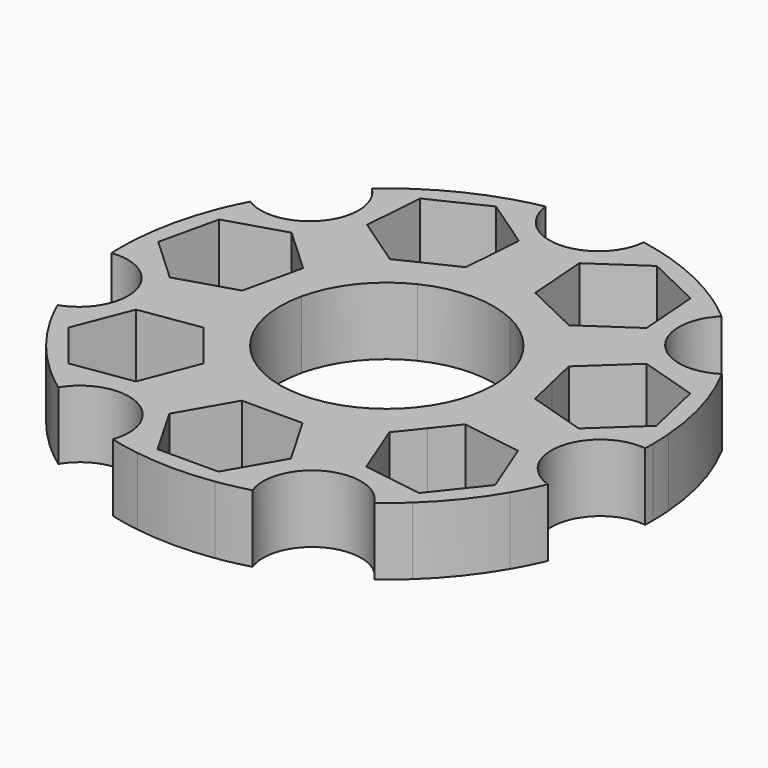
from build123d import *

# Parameters (mm, degrees)
F1_DEPTH = 6.9977
F4_D     = 10.16


# Not quite as in the source:
# - a feature names something its author has since deleted; it is built from what else it names


with BuildPart() as f1:
    # F0 (on Top) → F1 (new body)
    with BuildSketch(Plane.XY):
        with BuildLine():
            Line((13.000663339, 2.9673182751), (10.80089488, 2.4652351906))
            ThreePointArc((10.80089488, 2.4652351906), (11.0089999639, 1.2404170862), (11.0786603321, 0))
            ThreePointArc((11.0786603321, 0), (10.4569630833, -3.65904876), (8.6616464645, -6.9074304395))
            Line((8.6616464645, -6.9074304395), (10.4257240625, -8.3142349481))
            Line((10.4257240625, -8.3142349481), (12.9401280453, -5.1612711132))
            Line((12.9401280453, -5.1612711132), (20.9156255847, -6.3633827272))
            Line((20.9156255847, -6.3633827272), (23.8623151585, -13.8714220112))
            ThreePointArc((23.8623151585, -13.8714220112), (26.6500942722, -7.1832380314), (27.6012034762, 0))
            ThreePointArc((27.6012034762, 0), (27.5803414567, 1.0729391714), (27.5177869348, 2.1442564078))
            Line((27.5177869348, 2.1442564078), (21.6052967122, -3.3417341773))
            Line((21.6052967122, -3.3417341773), (13.8980443892, -0.9643627375))
            Line((13.8980443892, -0.9643627375), (13.000663339, 2.9673182751))
        make_face()
        with BuildLine():
            ThreePointArc((4.8068495738, 9.9815285367), (8.6616446562, 6.9074327071), (10.80089488, 2.4652351906))
            Line((10.80089488, 2.4652351906), (13.000663339, 2.9673182751))
            Line((13.000663339, 2.9673182751), (12.1032822888, 6.8989992876))
            Line((12.1032822888, 6.8989992876), (18.0157725115, 12.3849898727))
            Line((18.0157725115, 12.3849898727), (25.7230248345, 10.0076184329))
            ThreePointArc((25.7230248345, 10.0076184329), (21.5794879008, 17.2090713076), (15.4806129272, 22.8511937704))
            Line((15.4806129272, 22.8511937704), (16.0833555213, 14.8081635766))
            Line((16.0833555213, 14.8081635766), (9.419258347, 10.2646580813))
            Line((9.419258347, 10.2646580813), (5.7858384629, 12.0144204305))
            Line((5.7858384629, 12.0144204305), (4.8068495738, 9.9815285367))
        make_face()
        with BuildLine():
            Line((10.4257240625, -8.3142349481), (8.6616464645, -6.9074304395))
            ThreePointArc((8.6616464645, -6.9074304395), (4.8068513159, -9.9815276977), (0, -11.0786603321))
            Line((0, -11.0786603321), (0, -12.7))
            Line((0, -12.7), (0, -13.335))
            Line((0, -13.335), (4.0327916303, -13.335))
            Line((4.0327916303, -13.335), (8.0655832606, -20.32))
            Line((8.0655832606, -20.32), (4.0327916303, -27.305))
            ThreePointArc((4.0327916303, -27.305), (11.9757152285, -24.8678241529), (18.8335071928, -20.1773496811))
            Line((18.8335071928, -20.1773496811), (10.8580096534, -18.975238067))
            Line((10.8580096534, -18.975238067), (7.9113200797, -11.467198783))
            Line((7.9113200797, -11.467198783), (10.4257240625, -8.3142349481))
        make_face()
        with BuildLine():
            ThreePointArc((-4.8068513159, 9.9815276977), (-9.668e-07, 11.0786603321), (4.8068495738, 9.9815285367))
            Line((4.8068495738, 9.9815285367), (5.7858384629, 12.0144204305))
            Line((5.7858384629, 12.0144204305), (2.1524185788, 13.7641827798))
            Line((2.1524185788, 13.7641827798), (1.5496759847, 21.8072129736))
            Line((1.5496759847, 21.8072129736), (8.2137731589, 26.3507184689))
            ThreePointArc((8.2137731589, 26.3507184689), (-2.4087e-06, 27.6012034762), (-8.213777758, 26.3507170353))
            Line((-8.213777758, 26.3507170353), (-1.5496797908, 21.8072127031))
            Line((-1.5496797908, 21.8072127031), (-2.1524209811, 13.7641824041))
            Line((-2.1524209811, 13.7641824041), (-5.7858405598, 12.0144194207))
            Line((-5.7858405598, 12.0144194207), (-4.8068513159, 9.9815276977))
        make_face()
        Polygon((12.1032822888, 6.8989992876), (13.000663339, 2.9673182751), (13.8980443892, -0.9643627375), (21.6052967122, -3.3417341773), (27.5177869348, 2.1442564078), (25.7230248345, 10.0076184329), (18.0157725115, 12.3849898727), align=None)
        Polygon((15.188042256, 0.2325806629), (14.4864534349, 3.3064403636), (13.7848646139, 6.3803000643), (18.4073569698, 10.6693472491), (24.4330269677, 8.8106750325), (25.8362046098, 2.6629556311), (21.2137122539, -1.6260915537), align=None, mode=Mode.SUBTRACT)
        with BuildLine():
            Line((0, -12.7), (0, -11.0786603321))
            ThreePointArc((0, -11.0786603321), (-4.8068504449, -9.9815281172), (-8.661645259, -6.9074319513))
            Line((-8.661645259, -6.9074319513), (-10.4257226114, -8.3142367677))
            Line((-10.4257226114, -8.3142367677), (-7.9113180783, -11.4672001638))
            Line((-7.9113180783, -11.4672001638), (-10.8580063416, -18.9752399621))
            Line((-10.8580063416, -18.9752399621), (-18.8335036712, -20.1773529681))
            ThreePointArc((-18.8335036712, -20.1773529681), (-11.9757130584, -24.867825198), (-4.0327916303, -27.305))
            Line((-4.0327916303, -27.305), (-8.0655832606, -20.32))
            Line((-8.0655832606, -20.32), (-4.0327916303, -13.335))
            Line((-4.0327916303, -13.335), (0, -13.335))
            Line((0, -13.335), (0, -12.7))
        make_face()
        Polygon((12.9401280453, -5.1612711132), (10.4257240625, -8.3142349481), (7.9113200797, -11.467198783), (10.8580096534, -18.975238067), (18.8335071928, -20.1773496811), (23.8623151585, -13.8714220112), (20.9156255847, -6.3633827272), align=None)
        Polygon((9.6514286337, -11.7294776807), (11.6172353839, -9.2644332279), (13.5830421342, -6.7993887751), (19.8184311195, -7.7392214916), (22.1222066044, -13.6091431136), (18.190593104, -18.5392320191), (11.9552041187, -17.5993993027), align=None, mode=Mode.SUBTRACT)
        with BuildLine():
            ThreePointArc((-10.8008953103, 2.4652333055), (-8.6616458618, 6.9074311954), (-4.8068513159, 9.9815276977))
            Line((-4.8068513159, 9.9815276977), (-5.7858405598, 12.0144194207))
            Line((-5.7858405598, 12.0144194207), (-9.4192601386, 10.2646564373))
            Line((-9.4192601386, 10.2646564373), (-16.0833581058, 14.8081607695))
            Line((-16.0833581058, 14.8081607695), (-15.4806169155, 22.8511910685))
            ThreePointArc((-15.4806169155, 22.8511910685), (-21.5794909044, 17.2090675413), (-25.7230265811, 10.0076139433))
            Line((-25.7230265811, 10.0076139433), (-18.0157746731, 12.3849867284))
            Line((-18.0157746731, 12.3849867284), (-12.103283493, 6.8989971751))
            Line((-12.103283493, 6.8989971751), (-13.0006638569, 2.967316006))
            Line((-13.0006638569, 2.967316006), (-10.8008953103, 2.4652333055))
        make_face()
        Polygon((2.1524185788, 13.7641827798), (5.7858384629, 12.0144204305), (9.419258347, 10.2646580813), (16.0833555213, 14.8081635766), (15.4806129272, 22.8511937704), (8.2137731589, 26.3507184689), (1.5496759847, 21.8072129736), align=None)
        Polygon((9.287750872, 12.0195010326), (6.4470771444, 13.3874970511), (3.6064034168, 14.7554930697), (3.1351682978, 21.0436803121), (8.345280634, 24.5958755175), (14.0266280892, 21.8598834805), (14.4978632082, 15.5716962381), align=None, mode=Mode.SUBTRACT)
        with BuildLine():
            Line((-10.4257226114, -8.3142367677), (-8.661645259, -6.9074319513))
            ThreePointArc((-8.661645259, -6.9074319513), (-10.8008950951, -2.465234248), (-10.8008953103, 2.4652333055))
            Line((-10.8008953103, 2.4652333055), (-13.0006638569, 2.967316006))
            Line((-13.0006638569, 2.967316006), (-13.8980442209, -0.9643651631))
            Line((-13.8980442209, -0.9643651631), (-21.6052961289, -3.3417379482))
            Line((-21.6052961289, -3.3417379482), (-27.5177873091, 2.1442516051))
            ThreePointArc((-27.5177873091, 2.1442516051), (-26.909183449, -6.1418465822), (-23.8623127374, -13.8714261759))
            Line((-23.8623127374, -13.8714261759), (-20.9156244741, -6.3633863777))
            Line((-20.9156244741, -6.3633863777), (-12.9401271445, -5.1612733716))
            Line((-12.9401271445, -5.1612733716), (-10.4257226114, -8.3142367677))
        make_face()
        Polygon((-11.0835964967, -4.9326477372), (-9.8135964967, -7.1323522628), (-10.3635226281, -7.4498522628), (-11.6335226281, -5.2501477372), align=None, mode=Mode.SUBTRACT)
        Polygon((-9.4192601386, 10.2646564373), (-5.7858405598, 12.0144194207), (-2.1524209811, 13.7641824041), (-1.5496797908, 21.8072127031), (-8.213777758, 26.3507170353), (-15.4806169155, 22.8511910685), (-16.0833581058, 14.8081607695), align=None)
        Polygon((-3.6064059921, 14.7554924402), (-6.4470794809, 13.3874959259), (-9.2877529698, 12.0194994116), (-14.497865926, 15.5716937077), (-14.0266319045, 21.8598810324), (-8.3452849268, 24.595874061), (-3.1351719706, 21.0436797649), align=None, mode=Mode.SUBTRACT)
        Polygon((-7.9113180783, -11.4672001638), (-10.4257226114, -8.3142367677), (-12.9401271445, -5.1612733716), (-20.9156244741, -6.3633863777), (-23.8623127374, -13.8714261759), (-18.8335036712, -20.1773529681), (-10.8580063416, -18.9752399621), align=None)
        Polygon((-13.5830409474, -6.7993911458), (-11.617233767, -9.2644352555), (-9.6514265866, -11.7294793652), (-11.955201047, -17.5994013892), (-18.1905898683, -18.539235194), (-22.1222042292, -13.6091469746), (-19.8184297687, -7.7392249505), align=None, mode=Mode.SUBTRACT)
        Polygon((-13.8980442209, -0.9643651631), (-13.0006638569, 2.967316006), (-12.103283493, 6.8989971751), (-18.0157746731, 12.3849867284), (-25.7230265811, 10.0076139433), (-27.5177873091, 2.1442516051), (-21.6052961289, -3.3417379482), align=None)
        Polygon((-13.7848657274, 6.3802976584), (-14.486454012, 3.3064378353), (-15.1880422965, 0.2325780121), (-21.2137119701, -1.6260952562), (-25.8362050746, 2.6629511218), (-24.4330285055, 8.8106707681), (-18.4073588319, 10.6693440364), align=None, mode=Mode.SUBTRACT)
        Polygon((4.0327916303, -13.335), (0, -13.335), (-4.0327916303, -13.335), (-8.0655832606, -20.32), (-4.0327916303, -27.305), (4.0327916303, -27.305), (8.0655832606, -20.32), align=None)
        Polygon((-3.15290982, -14.859), (0, -14.859), (3.15290982, -14.859), (6.3058196401, -20.32), (3.15290982, -25.781), (-3.15290982, -25.781), (-6.3058196401, -20.32), align=None, mode=Mode.SUBTRACT)
        with BuildLine():
            Line((25.7230248345, 10.0076184329), (27.5177869348, 2.1442564078))
            ThreePointArc((27.5177869348, 2.1442564078), (26.9091829131, 6.1418489305), (25.7230248345, 10.0076184329))
        make_face()
        with BuildLine():
            Line((23.8623151585, -13.8714220112), (18.8335071928, -20.1773496811))
            ThreePointArc((18.8335071928, -20.1773496811), (21.5794924062, -17.2090656581), (23.8623151585, -13.8714220112))
        make_face()
        with BuildLine():
            Line((8.2137731589, 26.3507184689), (15.4806129272, 22.8511937704))
            ThreePointArc((15.4806129272, 22.8511937704), (11.9757108882, 24.8678262431), (8.2137731589, 26.3507184689))
        make_face()
        with BuildLine():
            ThreePointArc((-4.0327916303, -27.305), (0, -27.6012034762), (4.0327916303, -27.305))
            Line((4.0327916303, -27.305), (-4.0327916303, -27.305))
        make_face()
        with BuildLine():
            Line((-15.4806169155, 22.8511910685), (-8.213777758, 26.3507170353))
            ThreePointArc((-8.213777758, 26.3507170353), (-11.9757152285, 24.8678241529), (-15.4806169155, 22.8511910685))
        make_face()
        with BuildLine():
            Line((-18.8335036712, -20.1773529681), (-23.8623127374, -13.8714261759))
            ThreePointArc((-23.8623127374, -13.8714261759), (-21.5794894026, -17.2090694245), (-18.8335036712, -20.1773529681))
        make_face()
        with BuildLine():
            Line((-27.5177873091, 2.1442516051), (-25.7230265811, 10.0076139433))
            ThreePointArc((-25.7230265811, 10.0076139433), (-26.909183985, 6.141844234), (-27.5177873091, 2.1442516051))
        make_face()
        Polygon((-10.3635226281, -7.4498522628), (-9.8135964967, -7.1323522628), (-11.0835964967, -4.9326477372), (-11.6335226281, -5.2501477372), align=None)
    extrude(amount=F1_DEPTH)

    # F4 (through all)
    with Locations(Plane.XY.offset(6.9977)):
        with Locations((-21.6878161621, 17.115694081), (-0.1405437248, 27.6276781728), (21.5125610038, 17.3354570985), (26.9662685203, -6.0107167498), (12.1138258294, -24.8306982893), (-11.8605747881, -24.952657563), (-26.9037206785, -6.2847567503)):
            Hole(F4_D / 2)


solid = f1.part
